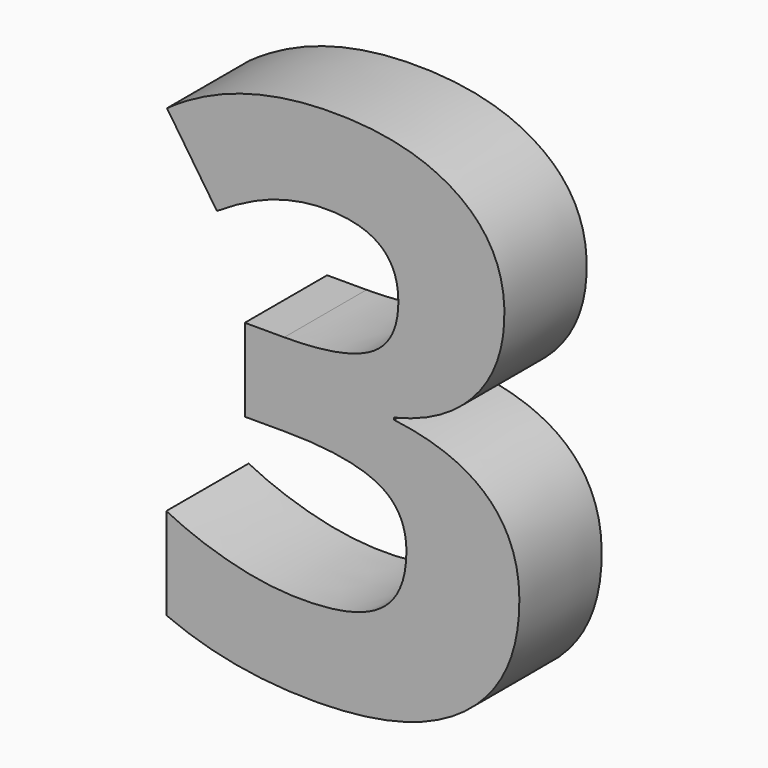
from build123d import *

# Parameters (mm, degrees)
F0_TEXT_SIZE = 35.2777777778
F1_DEPTH     = 5.08


# Not quite as in the source:
# - Text() gives the source's letters only with a copy of the font that has no kerning and outlines rounded to 1/6400 em; it was checked with that copy


with BuildPart() as f1:
    # F0 (on Front) → F1 (new body)
    with BuildSketch(Plane.XZ):
        with Locations((-14.9477215694, 2.5405713983)):
            Text('3', F0_TEXT_SIZE, font='Open Sans', font_style=FontStyle.BOLD, text_align=(TextAlign.LEFT, TextAlign.BOTTOM))
    extrude(amount=F1_DEPTH)


solid = f1.part
